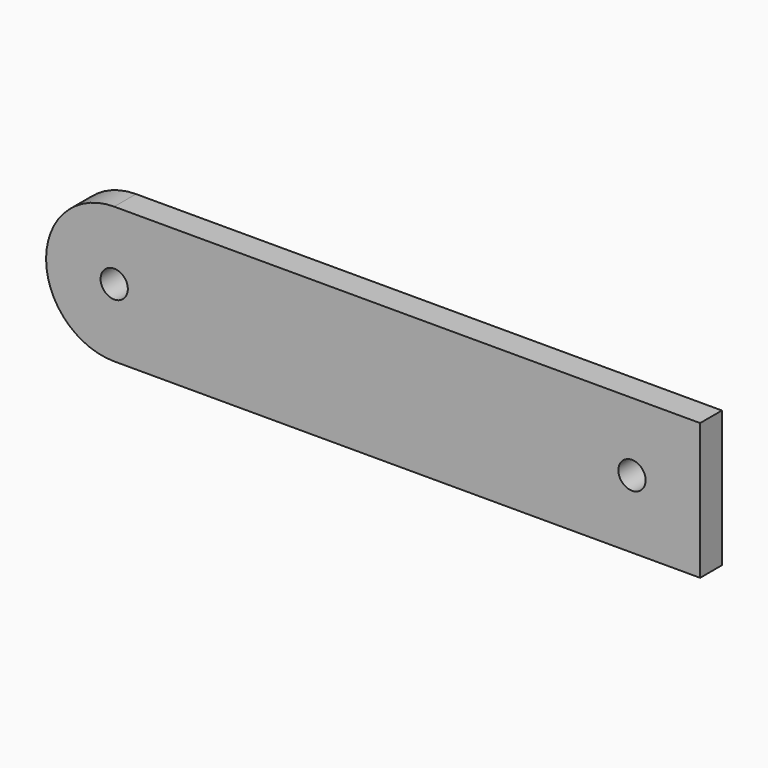
from build123d import *

# Parameters (mm, degrees)
F0_W     = 48
F0_H     = 10
F0_R     = 1
F1_DEPTH = 2
F2_R     = 4.99999


# Not quite as in the source:
# - a fillet or chamfer is up to 0.001 mm smaller than in the source, because OpenCascade refuses the exact size


with BuildPart() as f1:
    # F0 (on Front) → F1 (new body)
    with BuildSketch(Plane.XZ):
        with Locations((24, -5)):
            Rectangle(F0_W, F0_H)
        with Locations((5, -5)):
            Circle(F0_R, mode=Mode.SUBTRACT)
        with Locations((43, -5)):
            Circle(F0_R, mode=Mode.SUBTRACT)
    extrude(amount=F1_DEPTH)

    # F2 (radius 5 in the source; OpenCascade refuses exactly that, so slightly less here)
    f2_edges = [f1.edges().sort_by_distance(p)[0] for p in [
        (0, -1, 0),
        (0, -1, -10),
    ]]
    fillet(f2_edges, radius=F2_R)


solid = f1.part
